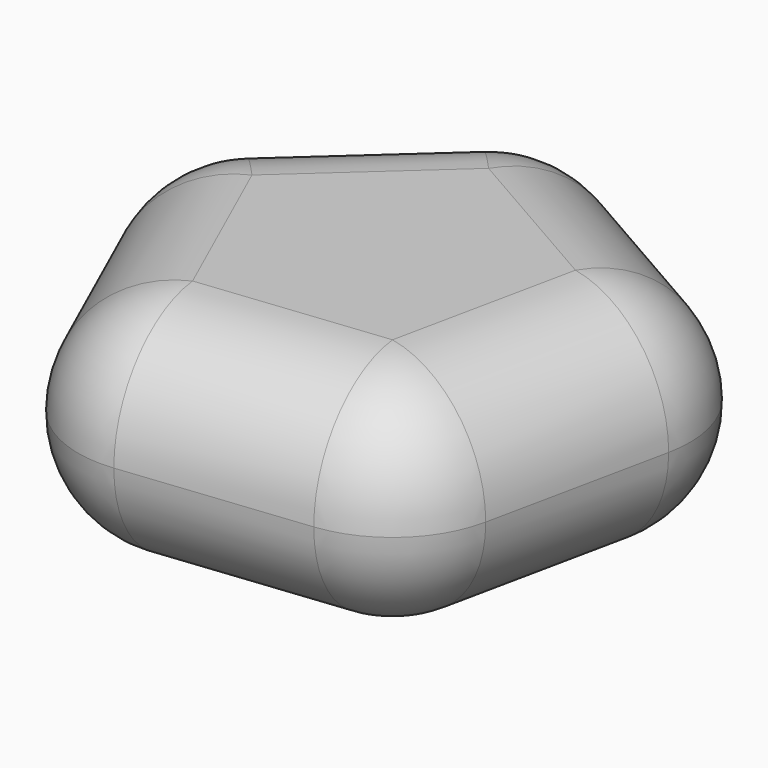
from build123d import *

# Parameters (mm, degrees)
F1_DEPTH = 25.4
F2_R     = 12.69999


# Not quite as in the source:
# - a fillet or chamfer is up to 0.001 mm smaller than in the source, because OpenCascade refuses the exact size


with BuildPart() as f1:
    # F0 (on Top) → F1 (new body)
    with BuildSketch(Plane.XY):
        Polygon((30.2693974938, 13.5768103187), (-3.5585556891, 32.9833728487), (-32.4687058605, 6.8080351654), (-16.5082081035, -28.7757757199), (22.2660721592, -24.5924426129), align=None)
    extrude(amount=F1_DEPTH)

    # F2 (radius 12.7 in the source; OpenCascade refuses exactly that, so slightly less here)
    f2_edges = [f1.edges().sort_by_distance(p)[0] for p in [
        (-16.508208, -28.775776, 12.7),
        (22.266072, -24.592443, 12.7),
        (2.878932, -26.684109, 0),
        (2.878932, -26.684109, 25.4),
        (-32.468706, 6.808035, 12.7),
        (-24.488457, -10.98387, 0),
        (-24.488457, -10.98387, 25.4),
        (-3.558556, 32.983373, 12.7),
        (-18.013631, 19.895704, 0),
        (-18.013631, 19.895704, 25.4),
        (30.269397, 13.57681, 12.7),
        (13.355421, 23.280092, 0),
        (13.355421, 23.280092, 25.4),
        (26.267735, -5.507816, 0),
        (26.267735, -5.507816, 25.4),
    ]]
    fillet(f2_edges, radius=F2_R)


solid = f1.part
